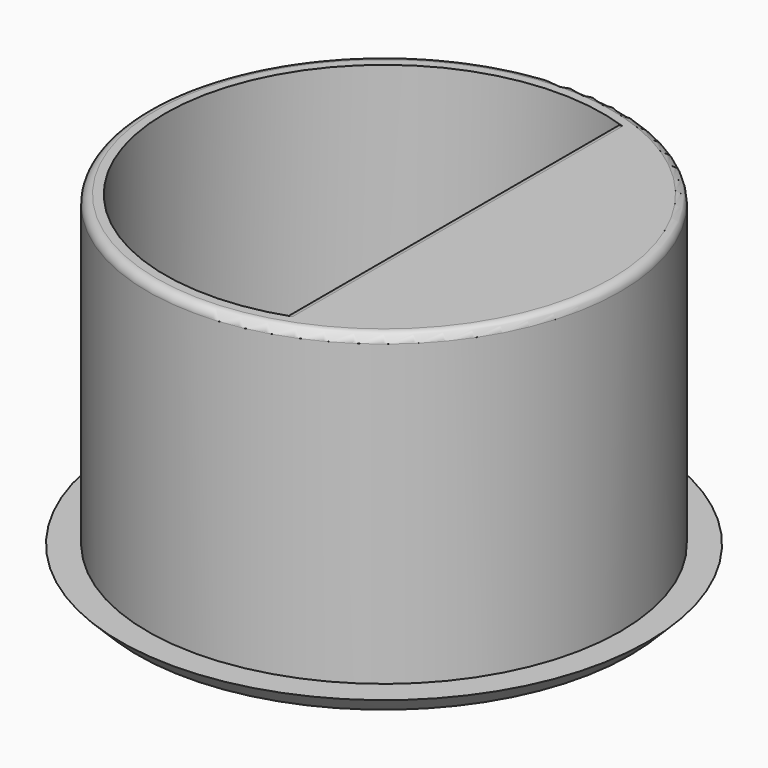
from build123d import *

# Parameters (mm, degrees)
F0_R     = 26.875
F0_R_2   = 24.875
F1_DEPTH = 37
F0_R_3   = 30
F2_DEPTH = 2
F4_DEPTH = 3
F5_R     = 1
F6_SIZE  = 1.99999


# Not quite as in the source:
# - a fillet or chamfer is up to 0.001 mm smaller than in the source, because OpenCascade refuses the exact size


with BuildPart() as f1:
    # F0 (on Top) → F1 (new body)
    with BuildSketch(Plane.XY):
        Circle(F0_R)
        Circle(F0_R_2, mode=Mode.SUBTRACT)
    extrude(amount=F1_DEPTH)

    # F0 (on Top) → F2 (join)
    with BuildSketch(Plane.XY):
        Circle(F0_R_3)
        Circle(F0_R, mode=Mode.SUBTRACT)
        Circle(F0_R_2)
    extrude(amount=F2_DEPTH)

    # F3 (on face) → F4 (join)
    with BuildSketch(Plane.XY.offset(37)):
        with BuildLine():
            ThreePointArc((7.3629554948, -23.7603137896), (20.0239749167, -14.7582537427), (24.875, 0))
            ThreePointArc((24.875, 0), (20.0239749167, 14.7582537427), (7.3629554948, 23.7603137896))
            Line((7.3629554948, 23.7603137896), (7.3629554948, -23.7603137896))
        make_face()
    extrude(amount=-F4_DEPTH)

    # F5
    f5_edges = [f1.edges().sort_by_distance(p)[0] for p in [
        (7.362955, 0, 34),
        (7.362955, 0, 37),
        (-26.875, 0, 37),
    ]]
    fillet(f5_edges, radius=F5_R)

    # F6 (size 2 in the source; OpenCascade refuses exactly that, so slightly less here)
    f6_edges = [f1.edges().sort_by_distance(p)[0] for p in [
        (-30, 0, 0),
    ]]
    chamfer(f6_edges, length=F6_SIZE)


solid = f1.part
